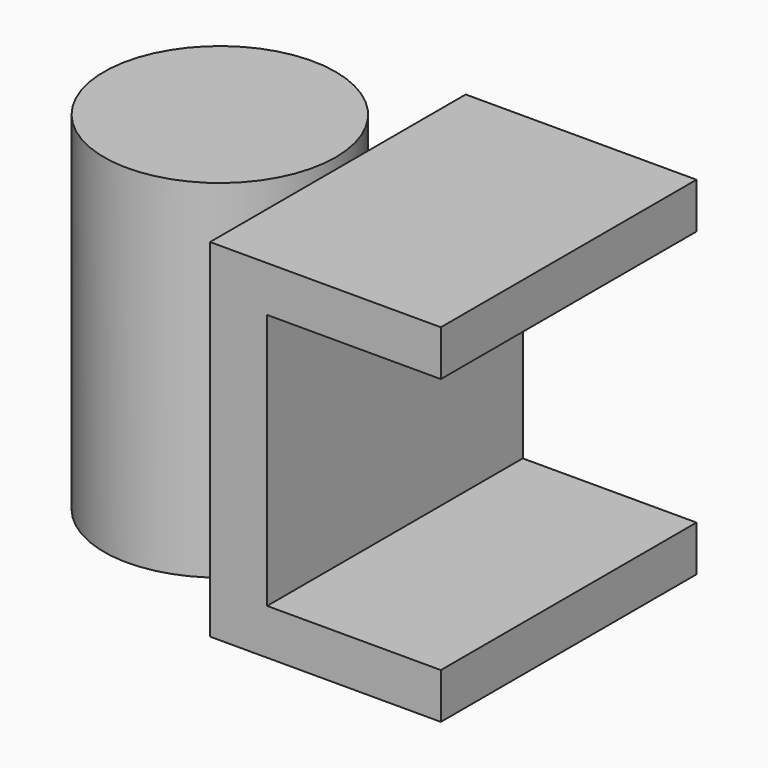
from build123d import *

# Parameters (mm, degrees)
F0_W     = 3.9854018639
F0_H     = 5.5182484599
F1_DEPTH = 6
F0_R     = 2
F4_W     = 5.5182484599
F4_H     = 4.4237960246
F5_DEPTH = 3


# Not quite as in the source:
# - a feature of the source that left no trace in its solid (it failed there, or was rolled back) is left out


with BuildPart() as f1:
    # F0 (on Top) → F1 (new body)
    with BuildSketch(Plane.XY):
        with Locations((4.2153283333, -0.2299270127)):
            Rectangle(F0_W, F0_H)
    extrude(amount=F1_DEPTH)

    # F4 (on face) → F5 (cut)
    with BuildSketch(Plane.YZ.offset(6.2080292652)):
        with Locations((-0.2299270127, 3.0000001134)):
            Rectangle(F4_W, F4_H)
    extrude(amount=-F5_DEPTH, mode=Mode.SUBTRACT)


with BuildPart() as f1b:
    # F0 (on Top) → F1, piece 2 (new body)
    with BuildSketch(Plane.XY):
        Circle(F0_R)
    extrude(amount=F1_DEPTH)


solid = Compound([f1.part, f1b.part])
